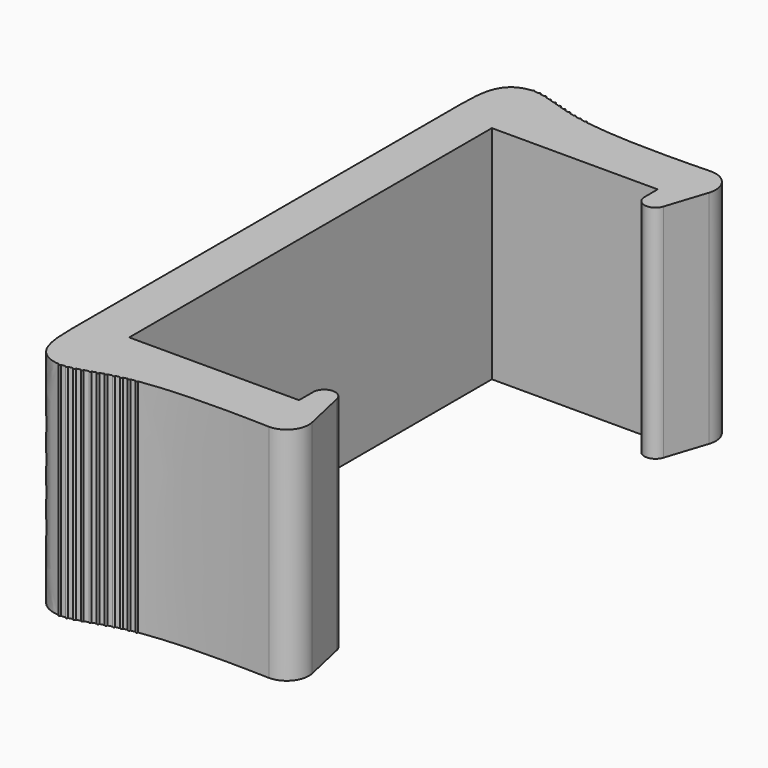
from build123d import *

# Parameters (mm, degrees)
F1_DEPTH = 10


with BuildPart() as f1:
    # F0 (on Top) → F1 (new body)
    with BuildSketch(Plane.XY):
        with BuildLine():
            add(Edge.make_bspline(
                [(-6, 11), (-5.9970486909, 11.7636909708), (-5.9267124346, 12.9377007904), (-5.0860900805, 13.3658969005), (-4.6793339712, 13.3827062938)],
                knots=[0, 0, 0, 0, 0.2094161864, 0.3671570668, 0.3671570668, 0.3671570668, 0.3671570668], degree=3))
            Line((-6, 11), (-6, -11))
            add(Edge.make_bspline(
                [(-6, -11), (-5.9970486909, -11.7636909708), (-5.9267124346, -12.9377007904), (-5.0860900805, -13.3658969005), (-4.6793339712, -13.3827062938)],
                knots=[0, 0, 0, 0, 0.2094161864, 0.3671570668, 0.3671570668, 0.3671570668, 0.3671570668], degree=3))
            add(Edge.make_bspline(
                [(-4.6793339712, -13.3827062938), (-4.6627459278, -13.3833918027), (-4.6295547085, -13.3842034837), (-4.5960885956, -13.3839043266), (-4.5793507778, -13.3834900812)],
                knots=[0.3671570668, 0.3671570668, 0.3671570668, 0.3671570668, 0.3735899451, 0.3799701109, 0.3799701109, 0.3799701109, 0.3799701109], degree=3))
            add(Edge.make_bspline(
                [(-4.5793507778, -13.3834900812), (-4.5137492525, -13.3818665042), (-4.447017118, -13.3761678251), (-4.3788267501, -13.3670049555)],
                knots=[0.3799701109, 0.3799701109, 0.3799701109, 0.3799701109, 0.4049762741, 0.4049762741, 0.4049762741, 0.4049762741], degree=3))
            add(Edge.make_bspline(
                [(-4.3788267501, -13.3670049555), (-4.3462400472, -13.3626262182), (-4.3133203309, -13.3574563716), (-4.2800318468, -13.3515620856)],
                knots=[0.4049762741, 0.4049762741, 0.4049762741, 0.4049762741, 0.416926179, 0.416926179, 0.416926179, 0.416926179], degree=3))
            add(Edge.make_bspline(
                [(-4.2800318468, -13.3515620856), (-4.2162228319, -13.3402636264), (-4.1510588491, -13.326303351), (-4.0842880773, -13.3101508235)],
                knots=[0.416926179, 0.416926179, 0.416926179, 0.416926179, 0.4398323486, 0.4398323486, 0.4398323486, 0.4398323486], degree=3))
            add(Edge.make_bspline(
                [(-4.0842880773, -13.3101508235), (-4.0523583298, -13.3024266934), (-4.0200611503, -13.2942012507), (-3.9873690016, -13.2855258431)],
                knots=[0.4398323486, 0.4398323486, 0.4398323486, 0.4398323486, 0.4507860667, 0.4507860667, 0.4507860667, 0.4507860667], degree=3))
            add(Edge.make_bspline(
                [(-3.9873690016, -13.2855258431), (-3.9246382724, -13.2688791967), (-3.8604533002, -13.2505758181), (-3.7946195353, -13.2309784783)],
                knots=[0.4507860667, 0.4507860667, 0.4507860667, 0.4507860667, 0.4718044074, 0.4718044074, 0.4718044074, 0.4718044074], degree=3))
            add(Edge.make_bspline(
                [(-3.7946195353, -13.2309784783), (-3.7632564746, -13.2216423487), (-3.7315192124, -13.2120125484), (-3.6993867139, -13.2021283004)],
                knots=[0.4718044074, 0.4718044074, 0.4718044074, 0.4718044074, 0.4818174986, 0.4818174986, 0.4818174986, 0.4818174986], degree=3))
            add(Edge.make_bspline(
                [(-3.6993867139, -13.2021283004), (-3.6372258613, -13.1830070584), (-3.5735858942, -13.1629335829), (-3.5083145277, -13.1421918355)],
                knots=[0.4818174986, 0.4818174986, 0.4818174986, 0.4818174986, 0.5011879902, 0.5011879902, 0.5011879902, 0.5011879902], degree=3))
            add(Edge.make_bspline(
                [(-3.5083145277, -13.1421918355), (-3.4769357527, -13.1322203785), (-3.4451799382, -13.1220944743), (-3.4130301643, -13.111845673)],
                knots=[0.5011879902, 0.5011879902, 0.5011879902, 0.5011879902, 0.5105002251, 0.5105002251, 0.5105002251, 0.5105002251], degree=3))
            add(Edge.make_bspline(
                [(-3.4130301643, -13.111845673), (-3.3509917517, -13.0920688819), (-3.2874863837, -13.0718344683), (-3.222392485, -13.0513691302)],
                knots=[0.5105002251, 0.5105002251, 0.5105002251, 0.5105002251, 0.5284697533, 0.5284697533, 0.5284697533, 0.5284697533], degree=3))
            add(Edge.make_bspline(
                [(-3.222392485, -13.0513691302), (-3.1909482676, -13.041483157), (-3.1591333724, -13.0315432983), (-3.1269340954, -13.0215751077)],
                knots=[0.5284697533, 0.5284697533, 0.5284697533, 0.5284697533, 0.5371501022, 0.5371501022, 0.5371501022, 0.5371501022], degree=3))
            add(Edge.make_bspline(
                [(-3.1269340954, -13.0215751077), (-3.0646065128, -13.0022798539), (-3.0008387027, -12.9828784438), (-2.9355312735, -12.96355621)],
                knots=[0.5371501022, 0.5371501022, 0.5371501022, 0.5371501022, 0.5539525032, 0.5539525032, 0.5539525032, 0.5539525032], degree=3))
            add(Edge.make_bspline(
                [(-2.9355312735, -12.96355621), (-2.9038965651, -12.9541965821), (-2.8719006001, -12.9448555322), (-2.8395320818, -12.9355541249)],
                knots=[0.5539525032, 0.5539525032, 0.5539525032, 0.5539525032, 0.5620915321, 0.5620915321, 0.5620915321, 0.5620915321], degree=3))
            add(Edge.make_bspline(
                [(-2.8395320818, -12.9355541249), (-2.7767266478, -12.917506375), (-2.7125186027, -12.8996078741), (-2.6468254236, -12.8820125007)],
                knots=[0.5620915321, 0.5620915321, 0.5620915321, 0.5620915321, 0.5778838906, 0.5778838906, 0.5778838906, 0.5778838906], degree=3))
            add(Edge.make_bspline(
                [(-2.6468254236, -12.8820125007), (-2.6149376531, -12.8734716257), (-2.5826999587, -12.8650021729), (-2.5501029025, -12.8566217414)],
                knots=[0.5778838906, 0.5778838906, 0.5778838906, 0.5778838906, 0.5855495739, 0.5855495739, 0.5855495739, 0.5855495739], degree=3))
            add(Edge.make_bspline(
                [(-2.5501029025, -12.8566217414), (-2.4867404351, -12.8403317791), (-2.4220201564, -12.8243781744), (-2.3558727479, -12.8088901834)],
                knots=[0.5855495739, 0.5855495739, 0.5855495739, 0.5855495739, 0.6004502018, 0.6004502018, 0.6004502018, 0.6004502018], degree=3))
            add(Edge.make_bspline(
                [(-2.3558727479, -12.8088901834), (-2.3237146214, -12.8013605645), (-2.2912191926, -12.7939409935), (-2.2583784966, -12.7866463223)],
                knots=[0.6004502018, 0.6004502018, 0.6004502018, 0.6004502018, 0.6076942691, 0.6076942691, 0.6076942691, 0.6076942691], degree=3))
            add(Edge.make_bspline(
                [(-2.2583784966, -12.7866463223), (-2.2010502926, -12.7739124145), (-2.1359549089, -12.7601382025), (-2.0694987676, -12.7469354112), (-2.0626289793, -12.7455795058)],
                knots=[0.6076942691, 0.6076942691, 0.6076942691, 0.6076942691, 0.6203398405, 0.6217943665, 0.6217943665, 0.6217943665, 0.6217943665], degree=3))
            add(Edge.make_bspline(
                [(-2.0626289793, -12.7455795058), (-2.0302056599, -12.7391800432), (-1.9974624251, -12.7329155042), (-1.964411746, -12.7267833983)],
                knots=[0.6217943665, 0.6217943665, 0.6217943665, 0.6217943665, 0.6286592883, 0.6286592883, 0.6286592883, 0.6286592883], degree=3))
            add(Edge.make_bspline(
                [(-1.964411746, -12.7267833983), (-1.8984355403, -12.7145424067), (-1.8312342101, -12.7028291434), (-1.7629069602, -12.6916237976)],
                knots=[0.6286592883, 0.6286592883, 0.6286592883, 0.6286592883, 0.6423631366, 0.6423631366, 0.6423631366, 0.6423631366], degree=3))
            add(Edge.make_bspline(
                [(-1.7629069602, -12.6916237976), (-1.7302421097, -12.6862669166), (-1.6973199348, -12.6810261181), (-1.6641512747, -12.6758992375)],
                knots=[0.6423631366, 0.6423631366, 0.6423631366, 0.6423631366, 0.6489144636, 0.6489144636, 0.6489144636, 0.6489144636], degree=3))
            add(Edge.make_bspline(
                [(-1.6641512747, -12.6758992375), (0.1133568257, -12.4011497686), (2.5987426278, -12.4535597596), (4.1238214885, -12.5)],
                knots=[0.6489144636, 0.6489144636, 0.6489144636, 0.6489144636, 1, 1, 1, 1], degree=3))
            ThreePointArc((4.1238214885, -12.5), (4.9044394426, -12.1250084877), (5.0996071824, -11.2812712193))
            Line((5.0996071824, -11.2812712193), (4.6751757339, -9.3878115006))
            ThreePointArc((4.6751757339, -9.3878115006), (4.123308576, -8.9559376665), (3.6816498572, -9.5000056261))
            Line((3.6816498572, -9.5000056261), (3.6780919435, -10.2499971869))
            Line((3.6780919435, -10.2499971869), (-4, -10.2499971869))
            Line((-4, -10.2499971869), (-4, 10.25))
            Line((-4, 10.25), (3.5, 10.25))
            Line((3.5, 10.25), (3.5, 9.5))
            ThreePointArc((3.5, 9.5), (3.9218174765, 9.0061503336), (4.475549972, 9.3455583473))
            Line((4.475549972, 9.3455583473), (5.0749214326, 11.1911166946))
            ThreePointArc((5.0749214326, 11.1911166946), (4.9327971696, 12.0878421109), (4.1238214885, 12.5))
            add(Edge.make_bspline(
                [(-1.6641512747, 12.6758992375), (0.1133568257, 12.4011497686), (2.5987426278, 12.4535597596), (4.1238214885, 12.5)],
                knots=[0.6489144636, 0.6489144636, 0.6489144636, 0.6489144636, 1, 1, 1, 1], degree=3))
            add(Edge.make_bspline(
                [(-1.7629069602, 12.6916237976), (-1.7302421097, 12.6862669166), (-1.6973199348, 12.6810261181), (-1.6641512747, 12.6758992375)],
                knots=[0.6423631366, 0.6423631366, 0.6423631366, 0.6423631366, 0.6489144636, 0.6489144636, 0.6489144636, 0.6489144636], degree=3))
            add(Edge.make_bspline(
                [(-1.964411746, 12.7267833983), (-1.8984355403, 12.7145424067), (-1.8312342101, 12.7028291434), (-1.7629069602, 12.6916237976)],
                knots=[0.6286592883, 0.6286592883, 0.6286592883, 0.6286592883, 0.6423631366, 0.6423631366, 0.6423631366, 0.6423631366], degree=3))
            add(Edge.make_bspline(
                [(-2.0626289793, 12.7455795058), (-2.0302056599, 12.7391800432), (-1.9974624251, 12.7329155042), (-1.964411746, 12.7267833983)],
                knots=[0.6217943665, 0.6217943665, 0.6217943665, 0.6217943665, 0.6286592883, 0.6286592883, 0.6286592883, 0.6286592883], degree=3))
            add(Edge.make_bspline(
                [(-2.2583784966, 12.7866463223), (-2.2010502926, 12.7739124145), (-2.1359549089, 12.7601382025), (-2.0694987676, 12.7469354112), (-2.0626289793, 12.7455795058)],
                knots=[0.6076942691, 0.6076942691, 0.6076942691, 0.6076942691, 0.6203398405, 0.6217943665, 0.6217943665, 0.6217943665, 0.6217943665], degree=3))
            add(Edge.make_bspline(
                [(-2.3558727479, 12.8088901834), (-2.3237146214, 12.8013605645), (-2.2912191926, 12.7939409935), (-2.2583784966, 12.7866463223)],
                knots=[0.6004502018, 0.6004502018, 0.6004502018, 0.6004502018, 0.6076942691, 0.6076942691, 0.6076942691, 0.6076942691], degree=3))
            add(Edge.make_bspline(
                [(-2.5501029025, 12.8566217414), (-2.4867404351, 12.8403317791), (-2.4220201564, 12.8243781744), (-2.3558727479, 12.8088901834)],
                knots=[0.5855495739, 0.5855495739, 0.5855495739, 0.5855495739, 0.6004502018, 0.6004502018, 0.6004502018, 0.6004502018], degree=3))
            add(Edge.make_bspline(
                [(-2.6468254236, 12.8820125007), (-2.6149376531, 12.8734716257), (-2.5826999587, 12.8650021729), (-2.5501029025, 12.8566217414)],
                knots=[0.5778838906, 0.5778838906, 0.5778838906, 0.5778838906, 0.5855495739, 0.5855495739, 0.5855495739, 0.5855495739], degree=3))
            add(Edge.make_bspline(
                [(-2.8395320818, 12.9355541249), (-2.7767266478, 12.917506375), (-2.7125186027, 12.8996078741), (-2.6468254236, 12.8820125007)],
                knots=[0.5620915321, 0.5620915321, 0.5620915321, 0.5620915321, 0.5778838906, 0.5778838906, 0.5778838906, 0.5778838906], degree=3))
            add(Edge.make_bspline(
                [(-2.9355312735, 12.96355621), (-2.9038965651, 12.9541965821), (-2.8719006001, 12.9448555322), (-2.8395320818, 12.9355541249)],
                knots=[0.5539525032, 0.5539525032, 0.5539525032, 0.5539525032, 0.5620915321, 0.5620915321, 0.5620915321, 0.5620915321], degree=3))
            add(Edge.make_bspline(
                [(-3.1269340954, 13.0215751077), (-3.0646065128, 13.0022798539), (-3.0008387027, 12.9828784438), (-2.9355312735, 12.96355621)],
                knots=[0.5371501022, 0.5371501022, 0.5371501022, 0.5371501022, 0.5539525032, 0.5539525032, 0.5539525032, 0.5539525032], degree=3))
            add(Edge.make_bspline(
                [(-3.222392485, 13.0513691302), (-3.1909482676, 13.041483157), (-3.1591333724, 13.0315432983), (-3.1269340954, 13.0215751077)],
                knots=[0.5284697533, 0.5284697533, 0.5284697533, 0.5284697533, 0.5371501022, 0.5371501022, 0.5371501022, 0.5371501022], degree=3))
            add(Edge.make_bspline(
                [(-3.4130301643, 13.111845673), (-3.3509917517, 13.0920688819), (-3.2874863837, 13.0718344683), (-3.222392485, 13.0513691302)],
                knots=[0.5105002251, 0.5105002251, 0.5105002251, 0.5105002251, 0.5284697533, 0.5284697533, 0.5284697533, 0.5284697533], degree=3))
            add(Edge.make_bspline(
                [(-3.5083145277, 13.1421918355), (-3.4769357527, 13.1322203785), (-3.4451799382, 13.1220944743), (-3.4130301643, 13.111845673)],
                knots=[0.5011879902, 0.5011879902, 0.5011879902, 0.5011879902, 0.5105002251, 0.5105002251, 0.5105002251, 0.5105002251], degree=3))
            add(Edge.make_bspline(
                [(-3.6993867139, 13.2021283004), (-3.6372258613, 13.1830070584), (-3.5735858942, 13.1629335829), (-3.5083145277, 13.1421918355)],
                knots=[0.4818174986, 0.4818174986, 0.4818174986, 0.4818174986, 0.5011879902, 0.5011879902, 0.5011879902, 0.5011879902], degree=3))
            add(Edge.make_bspline(
                [(-3.7946195353, 13.2309784783), (-3.7632564746, 13.2216423487), (-3.7315192124, 13.2120125484), (-3.6993867139, 13.2021283004)],
                knots=[0.4718044074, 0.4718044074, 0.4718044074, 0.4718044074, 0.4818174986, 0.4818174986, 0.4818174986, 0.4818174986], degree=3))
            add(Edge.make_bspline(
                [(-3.9873690016, 13.2855258431), (-3.9246382724, 13.2688791967), (-3.8604533002, 13.2505758181), (-3.7946195353, 13.2309784783)],
                knots=[0.4507860667, 0.4507860667, 0.4507860667, 0.4507860667, 0.4718044074, 0.4718044074, 0.4718044074, 0.4718044074], degree=3))
            add(Edge.make_bspline(
                [(-4.0842880773, 13.3101508235), (-4.0523583298, 13.3024266934), (-4.0200611503, 13.2942012507), (-3.9873690016, 13.2855258431)],
                knots=[0.4398323486, 0.4398323486, 0.4398323486, 0.4398323486, 0.4507860667, 0.4507860667, 0.4507860667, 0.4507860667], degree=3))
            add(Edge.make_bspline(
                [(-4.2800318468, 13.3515620856), (-4.2162228319, 13.3402636264), (-4.1510588491, 13.326303351), (-4.0842880773, 13.3101508235)],
                knots=[0.416926179, 0.416926179, 0.416926179, 0.416926179, 0.4398323486, 0.4398323486, 0.4398323486, 0.4398323486], degree=3))
            add(Edge.make_bspline(
                [(-4.3788267501, 13.3670049555), (-4.3462400472, 13.3626262182), (-4.3133203309, 13.3574563716), (-4.2800318468, 13.3515620856)],
                knots=[0.4049762741, 0.4049762741, 0.4049762741, 0.4049762741, 0.416926179, 0.416926179, 0.416926179, 0.416926179], degree=3))
            add(Edge.make_bspline(
                [(-4.5793507778, 13.3834900812), (-4.5137492525, 13.3818665042), (-4.447017118, 13.3761678251), (-4.3788267501, 13.3670049555)],
                knots=[0.3799701109, 0.3799701109, 0.3799701109, 0.3799701109, 0.4049762741, 0.4049762741, 0.4049762741, 0.4049762741], degree=3))
            add(Edge.make_bspline(
                [(-4.6793339712, 13.3827062938), (-4.6627459278, 13.3833918027), (-4.6295547085, 13.3842034837), (-4.5960885956, 13.3839043266), (-4.5793507778, 13.3834900812)],
                knots=[0.3671570668, 0.3671570668, 0.3671570668, 0.3671570668, 0.3735899451, 0.3799701109, 0.3799701109, 0.3799701109, 0.3799701109], degree=3))
        make_face()
        with BuildLine():
            ThreePointArc((-4.5793507778, 13.3834900812), (-4.6297408179, 13.4339252875), (-4.6793339712, 13.3827062938))
            add(Edge.make_bspline(
                [(-4.6793339712, 13.3827062938), (-4.6627459278, 13.3833918027), (-4.6295547085, 13.3842034837), (-4.5960885956, 13.3839043266), (-4.5793507778, 13.3834900812)],
                knots=[0.3671570668, 0.3671570668, 0.3671570668, 0.3671570668, 0.3735899451, 0.3799701109, 0.3799701109, 0.3799701109, 0.3799701109], degree=3))
        make_face()
        with BuildLine():
            add(Edge.make_bspline(
                [(-4.6793339712, -13.3827062938), (-4.6627459278, -13.3833918027), (-4.6295547085, -13.3842034837), (-4.5960885956, -13.3839043266), (-4.5793507778, -13.3834900812)],
                knots=[0.3671570668, 0.3671570668, 0.3671570668, 0.3671570668, 0.3735899451, 0.3799701109, 0.3799701109, 0.3799701109, 0.3799701109], degree=3))
            ThreePointArc((-4.6793339712, -13.3827062938), (-4.6297408179, -13.4339252875), (-4.5793507778, -13.3834900812))
        make_face()
        with BuildLine():
            ThreePointArc((-4.2800318468, 13.3515620856), (-4.3216270165, 13.409198186), (-4.3788267501, 13.3670049555))
            add(Edge.make_bspline(
                [(-4.3788267501, 13.3670049555), (-4.3462400472, 13.3626262182), (-4.3133203309, 13.3574563716), (-4.2800318468, 13.3515620856)],
                knots=[0.4049762741, 0.4049762741, 0.4049762741, 0.4049762741, 0.416926179, 0.416926179, 0.416926179, 0.416926179], degree=3))
        make_face()
        with BuildLine():
            add(Edge.make_bspline(
                [(-4.3788267501, -13.3670049555), (-4.3462400472, -13.3626262182), (-4.3133203309, -13.3574563716), (-4.2800318468, -13.3515620856)],
                knots=[0.4049762741, 0.4049762741, 0.4049762741, 0.4049762741, 0.416926179, 0.416926179, 0.416926179, 0.416926179], degree=3))
            ThreePointArc((-4.3788267501, -13.3670049555), (-4.3216270165, -13.409198186), (-4.2800318468, -13.3515620856))
        make_face()
        with BuildLine():
            ThreePointArc((-3.9873690016, 13.2855258431), (-4.0234480756, 13.3465654022), (-4.0842880773, 13.3101508235))
            add(Edge.make_bspline(
                [(-4.0842880773, 13.3101508235), (-4.0523583298, 13.3024266934), (-4.0200611503, 13.2942012507), (-3.9873690016, 13.2855258431)],
                knots=[0.4398323486, 0.4398323486, 0.4398323486, 0.4398323486, 0.4507860667, 0.4507860667, 0.4507860667, 0.4507860667], degree=3))
        make_face()
        with BuildLine():
            add(Edge.make_bspline(
                [(-4.0842880773, -13.3101508235), (-4.0523583298, -13.3024266934), (-4.0200611503, -13.2942012507), (-3.9873690016, -13.2855258431)],
                knots=[0.4398323486, 0.4398323486, 0.4398323486, 0.4398323486, 0.4507860667, 0.4507860667, 0.4507860667, 0.4507860667], degree=3))
            ThreePointArc((-4.0842880773, -13.3101508235), (-4.0234480756, -13.3465654022), (-3.9873690016, -13.2855258431))
        make_face()
        with BuildLine():
            ThreePointArc((-3.6993867139, 13.2021283004), (-3.7339443978, 13.2596595153), (-3.7946195353, 13.2309784783))
            add(Edge.make_bspline(
                [(-3.7946195353, 13.2309784783), (-3.7632564746, 13.2216423487), (-3.7315192124, 13.2120125484), (-3.6993867139, 13.2021283004)],
                knots=[0.4718044074, 0.4718044074, 0.4718044074, 0.4718044074, 0.4818174986, 0.4818174986, 0.4818174986, 0.4818174986], degree=3))
        make_face()
        with BuildLine():
            add(Edge.make_bspline(
                [(-3.7946195353, -13.2309784783), (-3.7632564746, -13.2216423487), (-3.7315192124, -13.2120125484), (-3.6993867139, -13.2021283004)],
                knots=[0.4718044074, 0.4718044074, 0.4718044074, 0.4718044074, 0.4818174986, 0.4818174986, 0.4818174986, 0.4818174986], degree=3))
            ThreePointArc((-3.7946195353, -13.2309784783), (-3.7339443978, -13.2596595153), (-3.6993867139, -13.2021283004))
        make_face()
        with BuildLine():
            ThreePointArc((-3.4130301643, 13.111845673), (-3.4454958249, 13.1746717367), (-3.5083145277, 13.1421918355))
            add(Edge.make_bspline(
                [(-3.5083145277, 13.1421918355), (-3.4769357527, 13.1322203785), (-3.4451799382, 13.1220944743), (-3.4130301643, 13.111845673)],
                knots=[0.5011879902, 0.5011879902, 0.5011879902, 0.5011879902, 0.5105002251, 0.5105002251, 0.5105002251, 0.5105002251], degree=3))
        make_face()
        with BuildLine():
            add(Edge.make_bspline(
                [(-3.5083145277, -13.1421918355), (-3.4769357527, -13.1322203785), (-3.4451799382, -13.1220944743), (-3.4130301643, -13.111845673)],
                knots=[0.5011879902, 0.5011879902, 0.5011879902, 0.5011879902, 0.5105002251, 0.5105002251, 0.5105002251, 0.5105002251], degree=3))
            ThreePointArc((-3.5083145277, -13.1421918355), (-3.4454958249, -13.1746717367), (-3.4130301643, -13.111845673))
        make_face()
        with BuildLine():
            ThreePointArc((-3.1269340954, 13.0215751077), (-3.1597826412, 13.0841488902), (-3.222392485, 13.0513691302))
            add(Edge.make_bspline(
                [(-3.222392485, 13.0513691302), (-3.1909482676, 13.041483157), (-3.1591333724, 13.0315432983), (-3.1269340954, 13.0215751077)],
                knots=[0.5284697533, 0.5284697533, 0.5284697533, 0.5284697533, 0.5371501022, 0.5371501022, 0.5371501022, 0.5371501022], degree=3))
        make_face()
        with BuildLine():
            add(Edge.make_bspline(
                [(-3.222392485, -13.0513691302), (-3.1909482676, -13.041483157), (-3.1591333724, -13.0315432983), (-3.1269340954, -13.0215751077)],
                knots=[0.5284697533, 0.5284697533, 0.5284697533, 0.5284697533, 0.5371501022, 0.5371501022, 0.5371501022, 0.5371501022], degree=3))
            ThreePointArc((-3.222392485, -13.0513691302), (-3.1597826412, -13.0841488902), (-3.1269340954, -13.0215751077))
        make_face()
        with BuildLine():
            ThreePointArc((-2.8395320818, 12.9355541249), (-2.8735580581, 12.9974607496), (-2.9355312735, 12.96355621))
            add(Edge.make_bspline(
                [(-2.9355312735, 12.96355621), (-2.9038965651, 12.9541965821), (-2.8719006001, 12.9448555322), (-2.8395320818, 12.9355541249)],
                knots=[0.5539525032, 0.5539525032, 0.5539525032, 0.5539525032, 0.5620915321, 0.5620915321, 0.5620915321, 0.5620915321], degree=3))
        make_face()
        with BuildLine():
            add(Edge.make_bspline(
                [(-2.9355312735, -12.96355621), (-2.9038965651, -12.9541965821), (-2.8719006001, -12.9448555322), (-2.8395320818, -12.9355541249)],
                knots=[0.5539525032, 0.5539525032, 0.5539525032, 0.5539525032, 0.5620915321, 0.5620915321, 0.5620915321, 0.5620915321], degree=3))
            ThreePointArc((-2.9355312735, -12.96355621), (-2.8735580581, -12.9974607496), (-2.8395320818, -12.9355541249))
        make_face()
        with BuildLine():
            ThreePointArc((-2.5501029025, 12.8566217414), (-2.5858006693, 12.9175569168), (-2.6468254236, 12.8820125007))
            add(Edge.make_bspline(
                [(-2.6468254236, 12.8820125007), (-2.6149376531, 12.8734716257), (-2.5826999587, 12.8650021729), (-2.5501029025, 12.8566217414)],
                knots=[0.5778838906, 0.5778838906, 0.5778838906, 0.5778838906, 0.5855495739, 0.5855495739, 0.5855495739, 0.5855495739], degree=3))
        make_face()
        with BuildLine():
            add(Edge.make_bspline(
                [(-2.6468254236, -12.8820125007), (-2.6149376531, -12.8734716257), (-2.5826999587, -12.8650021729), (-2.5501029025, -12.8566217414)],
                knots=[0.5778838906, 0.5778838906, 0.5778838906, 0.5778838906, 0.5855495739, 0.5855495739, 0.5855495739, 0.5855495739], degree=3))
            ThreePointArc((-2.6468254236, -12.8820125007), (-2.5858006693, -12.9175569168), (-2.5501029025, -12.8566217414))
        make_face()
        with BuildLine():
            ThreePointArc((-2.2583784966, 12.7866463223), (-2.2960354198, 12.8463763153), (-2.3558727479, 12.8088901834))
            add(Edge.make_bspline(
                [(-2.3558727479, 12.8088901834), (-2.3237146214, 12.8013605645), (-2.2912191926, 12.7939409935), (-2.2583784966, 12.7866463223)],
                knots=[0.6004502018, 0.6004502018, 0.6004502018, 0.6004502018, 0.6076942691, 0.6076942691, 0.6076942691, 0.6076942691], degree=3))
        make_face()
        with BuildLine():
            add(Edge.make_bspline(
                [(-2.3558727479, -12.8088901834), (-2.3237146214, -12.8013605645), (-2.2912191926, -12.7939409935), (-2.2583784966, -12.7866463223)],
                knots=[0.6004502018, 0.6004502018, 0.6004502018, 0.6004502018, 0.6076942691, 0.6076942691, 0.6076942691, 0.6076942691], degree=3))
            ThreePointArc((-2.3558727479, -12.8088901834), (-2.2960354198, -12.8463763153), (-2.2583784966, -12.7866463223))
        make_face()
        with BuildLine():
            ThreePointArc((-1.964411746, 12.7267833983), (-2.0041490902, 12.7851501253), (-2.0626289793, 12.7455795058))
            add(Edge.make_bspline(
                [(-2.0626289793, 12.7455795058), (-2.0302056599, 12.7391800432), (-1.9974624251, 12.7329155042), (-1.964411746, 12.7267833983)],
                knots=[0.6217943665, 0.6217943665, 0.6217943665, 0.6217943665, 0.6286592883, 0.6286592883, 0.6286592883, 0.6286592883], degree=3))
        make_face()
        with BuildLine():
            add(Edge.make_bspline(
                [(-2.0626289793, -12.7455795058), (-2.0302056599, -12.7391800432), (-1.9974624251, -12.7329155042), (-1.964411746, -12.7267833983)],
                knots=[0.6217943665, 0.6217943665, 0.6217943665, 0.6217943665, 0.6286592883, 0.6286592883, 0.6286592883, 0.6286592883], degree=3))
            ThreePointArc((-2.0626289793, -12.7455795058), (-2.0041490902, -12.7851501253), (-1.964411746, -12.7267833983))
        make_face()
        with BuildLine():
            ThreePointArc((-1.6641512747, 12.6758992375), (-1.7056848815, 12.7330260374), (-1.7629069602, 12.6916237976))
            add(Edge.make_bspline(
                [(-1.7629069602, 12.6916237976), (-1.7302421097, 12.6862669166), (-1.6973199348, 12.6810261181), (-1.6641512747, 12.6758992375)],
                knots=[0.6423631366, 0.6423631366, 0.6423631366, 0.6423631366, 0.6489144636, 0.6489144636, 0.6489144636, 0.6489144636], degree=3))
        make_face()
        with BuildLine():
            add(Edge.make_bspline(
                [(-1.7629069602, -12.6916237976), (-1.7302421097, -12.6862669166), (-1.6973199348, -12.6810261181), (-1.6641512747, -12.6758992375)],
                knots=[0.6423631366, 0.6423631366, 0.6423631366, 0.6423631366, 0.6489144636, 0.6489144636, 0.6489144636, 0.6489144636], degree=3))
            ThreePointArc((-1.7629069602, -12.6916237976), (-1.7056848815, -12.7330260374), (-1.6641512747, -12.6758992375))
        make_face()
    extrude(amount=F1_DEPTH)


solid = f1.part
